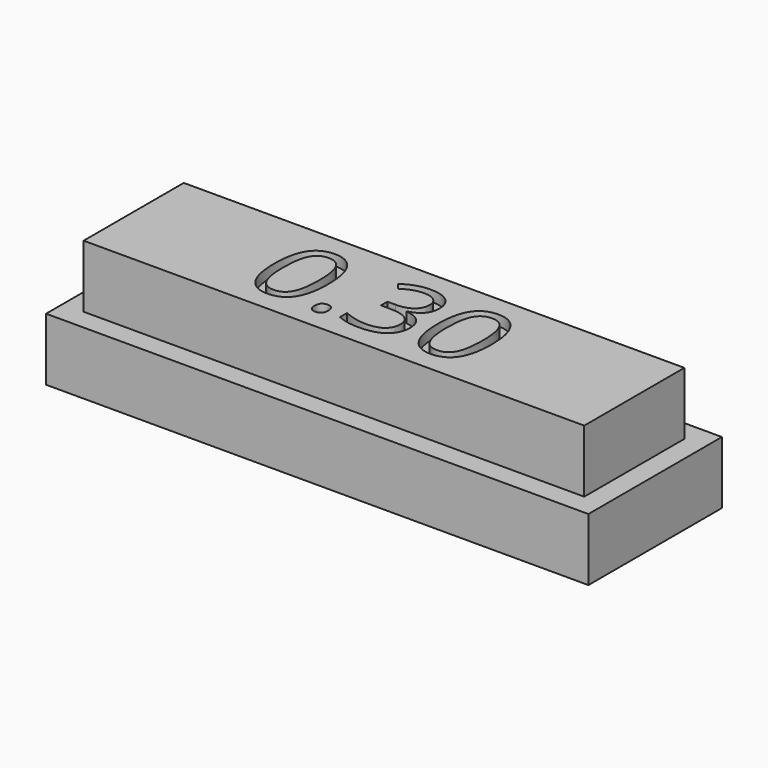
from build123d import *

# Parameters (mm, degrees)
F0_W         = 26
F0_H         = 8
F0_W_2       = 20
F0_H_2       = 2
F1_DEPTH     = 3
F2_W         = 24
F2_H         = 6
F3_DEPTH     = 3
F4_W         = 19.4
F4_H         = 1.4
F5_DEPTH     = 3
F5_TAPER     = 5
F6_TEXT_SIZE = 5.5555555556
F7_DEPTH     = 0.5


# Not quite as in the source:
# - Text() gives the source's letters only with a copy of the font that has no kerning and outlines rounded to 1/6400 em; it was checked with that copy


with BuildPart() as f1:
    # F0 (on Top) → F1 (new body)
    with BuildSketch(Plane.XY):
        Rectangle(F0_W, F0_H)
        Rectangle(F0_W_2, F0_H_2, mode=Mode.SUBTRACT)
    extrude(amount=F1_DEPTH)


with BuildPart() as f3:
    # F2 (on face) → F3 (new body)
    with BuildSketch(Plane.XY.offset(3)):
        Rectangle(F2_W, F2_H)
    extrude(amount=F3_DEPTH)

    # F4 (on face) → F5 (join, through all)
    with BuildSketch(Plane(origin=(0, 0, 3), x_dir=(1, 0, 0), z_dir=(0, 0, -1))):
        Rectangle(F4_W, F4_H)
    extrude(amount=F5_DEPTH, taper=F5_TAPER)

    # F6 (on face) → F7 (cut)
    with BuildSketch(Plane.XY.offset(6)):
        with Locations((-5.5455729167, -2)):
            Text('0.30', F6_TEXT_SIZE, font='Open Sans', text_align=(TextAlign.LEFT, TextAlign.BOTTOM))
    extrude(amount=-F7_DEPTH, mode=Mode.SUBTRACT)


solid = Compound([f1.part, f3.part])
